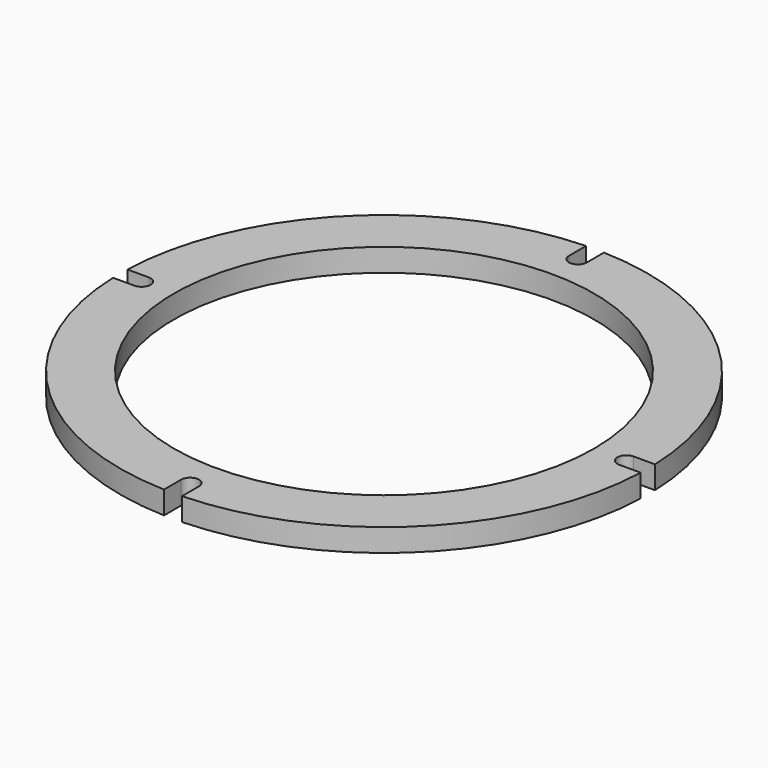
from build123d import *

# Parameters (mm, degrees)
F0_R     = 58.5
F1_DEPTH = 6.35


# Not quite as in the source:
# - a length typed as a fraction of an inch, garbled in the dataset ("3 / 203.2 mm" for 3/8 in), is restored


with BuildPart() as f1:
    # F0 (on Top) → F1 (new body)
    with BuildSketch(Plane.XY):
        with BuildLine():
            Line((67.5, 2.5), (73.4574706888, 2.5))
            ThreePointArc((73.4574706888, 2.5), (51.9723484172, 51.9723484172), (2.5, 73.4574706888))
            Line((2.5, 73.4574706888), (2.5, 67.5))
            ThreePointArc((2.5, 67.5), (0, 65), (-2.5, 67.5))
            Line((-2.5, 67.5), (-2.5, 73.4574706888))
            ThreePointArc((-2.5, 73.4574706888), (-51.9723484172, 51.9723484172), (-73.4574706888, 2.5))
            Line((-73.4574706888, 2.5), (-67.5, 2.5))
            ThreePointArc((-67.5, 2.5), (-65.732233047, 1.767766953), (-65, 0))
            ThreePointArc((-65, 0), (-65.732233047, -1.767766953), (-67.5, -2.5))
            Line((-67.5, -2.5), (-73.4574706888, -2.5))
            ThreePointArc((-73.4574706888, -2.5), (-51.9723484172, -51.9723484172), (-2.5, -73.4574706888))
            Line((-2.5, -73.4574706888), (-2.5, -67.5))
            ThreePointArc((-2.5, -67.5), (0, -65), (2.5, -67.5))
            Line((2.5, -67.5), (2.5, -73.4574706888))
            ThreePointArc((2.5, -73.4574706888), (51.9723484172, -51.9723484172), (73.4574706888, -2.5))
            Line((73.4574706888, -2.5), (67.5, -2.5))
            ThreePointArc((67.5, -2.5), (65, 0), (67.5, 2.5))
        make_face()
        Circle(F0_R, mode=Mode.SUBTRACT)
    extrude(amount=F1_DEPTH)


solid = f1.part
